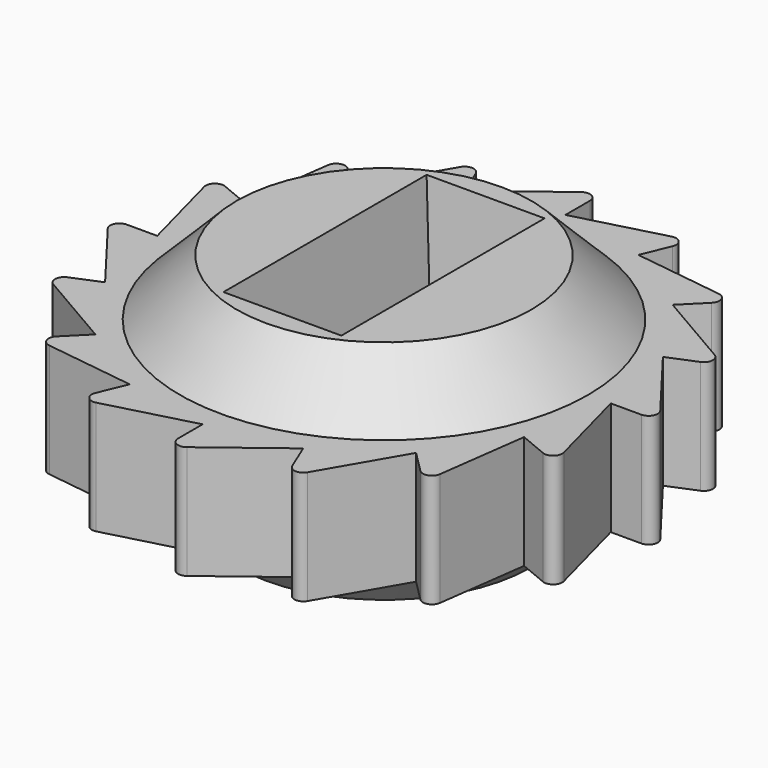
from build123d import *

# Parameters (mm, degrees)
F0_R       = 45
F0_W       = 20
F0_H       = 50
F1_DEPTH   = 12.5
F2_DEPTH   = 25
F3_SIZE2   = 12.49999
F3_SIZE    = 12.49999
F4_SIZE    = 12.49999
F5_R       = 2
F6_SIZE2   = 20
F6_SIZE    = 3
F6_2_SIZE2 = 20
F6_2_SIZE  = 3
F7_SIZE2   = 3
F7_SIZE    = 20


# Not quite as in the source:
# - a fillet or chamfer is up to 0.001 mm smaller than in the source, because OpenCascade refuses the exact size


with BuildPart() as f1:
    # F0 (on Top) → F1 (new body, symmetric)
    with BuildSketch(Plane.XY):
        Polygon((46.1939766256, -19.1341716183), (50, 0), (46.1939766256, 19.1341716183), (35.3553390593, 35.3553390593), (19.1341716183, 46.1939766256), (0, 50), (-19.1341716183, 46.1939766256), (-35.3553390593, 35.3553390593), (-46.1939766256, 19.1341716183), (-50, 0), (-46.1939766256, -19.1341716183), (-35.3553390593, -35.3553390593), (-19.1341716183, -46.1939766256), (0, -50), (19.1341716183, -46.1939766256), (35.3553390593, -35.3553390593), align=None)
        Circle(F0_R, mode=Mode.SUBTRACT)
        Circle(F0_R)
        Rectangle(F0_W, F0_H, mode=Mode.SUBTRACT)
        Polygon((-19.1341716183, 46.1939766256), (0, 50), (0, 60.7945092961), align=None)
        Polygon((-35.3553390593, 35.3553390593), (-19.1341716183, 46.1939766256), (-23.2650514864, 56.1668028277), align=None)
        Polygon((-46.1939766256, 19.1341716183), (-35.3553390593, 35.3553390593), (-42.9882097822, 42.9882097822), align=None)
        Polygon((-50, 0), (-46.1939766256, 19.1341716183), (-56.1668028277, 23.2650514864), align=None)
        Polygon((-60.7945092961, 0), (-46.1939766256, -19.1341716183), (-50, 0), align=None)
        Polygon((-56.1668028277, -23.2650514864), (-35.3553390593, -35.3553390593), (-46.1939766256, -19.1341716183), align=None)
        Polygon((-42.9882097822, -42.9882097822), (-19.1341716183, -46.1939766256), (-35.3553390593, -35.3553390593), align=None)
        Polygon((-23.2650514864, -56.1668028277), (0, -50), (-19.1341716183, -46.1939766256), align=None)
        Polygon((0, -60.7945092961), (19.1341716183, -46.1939766256), (0, -50), align=None)
        Polygon((23.2650514864, -56.1668028277), (35.3553390593, -35.3553390593), (19.1341716183, -46.1939766256), align=None)
        Polygon((42.9882097822, -42.9882097822), (46.1939766256, -19.1341716183), (35.3553390593, -35.3553390593), align=None)
        Polygon((56.1668028277, -23.2650514864), (50, 0), (46.1939766256, -19.1341716183), align=None)
        Polygon((46.1939766256, 19.1341716183), (50, 0), (60.7945092961, 0), align=None)
        Polygon((35.3553390593, 35.3553390593), (46.1939766256, 19.1341716183), (56.1668028277, 23.2650514864), align=None)
        Polygon((19.1341716183, 46.1939766256), (35.3553390593, 35.3553390593), (42.9882097822, 42.9882097822), align=None)
        Polygon((0, 50), (19.1341716183, 46.1939766256), (23.2650514864, 56.1668028277), align=None)
    extrude(amount=F1_DEPTH, both=True)

    # F0 (on Top) → F2 (join, symmetric)
    with BuildSketch(Plane.XY):
        Circle(F0_R)
        Rectangle(F0_W, F0_H, mode=Mode.SUBTRACT)
    extrude(amount=F2_DEPTH, both=True)

    # F3 (size 12.5 and 12.5 in the source; OpenCascade refuses exactly that, so slightly less here)
    f3_edges = [f1.edges().sort_by_distance(p)[0] for p in [
        (-45, 0, 25),
    ]]
    chamfer(f3_edges, length=F3_SIZE, length2=F3_SIZE2)

    # F4 (size 12.5 in the source; OpenCascade refuses exactly that, so slightly less here)
    f4_edges = [f1.edges().sort_by_distance(p)[0] for p in [
        (-45, 0, -25),
    ]]
    chamfer(f4_edges, length=F4_SIZE)

    # F5
    f5_edges = [f1.edges().sort_by_distance(p)[0] for p in [
        (23.265051, 56.166803, 0),
        (0, 60.794509, 0),
        (-23.265051, 56.166803, 0),
        (-42.98821, 42.98821, 0),
        (-56.166803, 23.265051, 0),
        (-60.794509, 0, 0),
        (-56.166803, -23.265051, 0),
        (-42.98821, -42.98821, 0),
        (-23.265051, -56.166803, 0),
        (0, -60.794509, 0),
        (23.265051, -56.166803, 0),
        (42.98821, 42.98821, 0),
        (56.166803, 23.265051, 0),
        (60.794509, 0, 0),
        (56.166803, -23.265051, 0),
        (42.98821, -42.98821, 0),
    ]]
    fillet(f5_edges, radius=F5_R)

    # F6
    f6_edges = [f1.edges().sort_by_distance(p)[0] for p in [
        (0, 25, -25),
        (-10, 0, -25),
        (10, 0, -25),
        (0, -25, -25),
    ]]
    f6_side = f1.faces().sort_by_distance((-31.580771, 0, -25))[0]
    chamfer(f6_edges, length=F6_SIZE, length2=F6_SIZE2, reference=f6_side)

    # F6#2
    f6_2_edges = [f1.edges().sort_by_distance(p)[0] for p in [
        (-10, 0, 25),
        (0, -25, 25),
        (0, 25, 25),
    ]]
    f6_2_side = f1.faces().sort_by_distance((-31.580771, 0, 25))[0]
    chamfer(f6_2_edges, length=F6_2_SIZE, length2=F6_2_SIZE2, reference=f6_2_side)

    # F7
    f7_edges = [f1.edges().sort_by_distance(p)[0] for p in [
        (10, 0, 25),
    ]]
    f7_side = f1.faces().sort_by_distance((10, 0, 10.320513))[0]
    chamfer(f7_edges, length=F7_SIZE, length2=F7_SIZE2, reference=f7_side)


solid = f1.part
